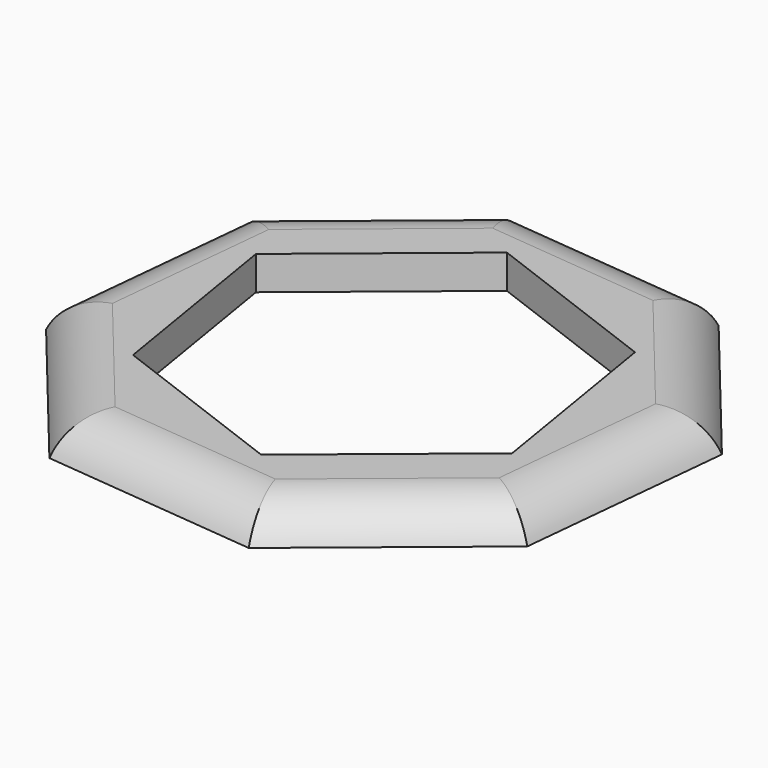
from build123d import *

# Parameters (mm, degrees)
F1_DEPTH     = 3
F2_T1_DEPTH  = 42.25719254
F2_T3_DEPTH  = 42.25719254
F2_T5_DEPTH  = 42.25719254
F2_T7_DEPTH  = 42.25719254
F2_T9_DEPTH  = 42.25719254
F2_T11_DEPTH = 42.25719254
F2_T13_DEPTH = 42.25719254
F2_T15_DEPTH = 42.25719254


# Not quite as in the source:
# - a fillet or chamfer that OpenCascade refuses, or shapes differently, is made with other operations: its cross-section is extruded or revolved along the edge and cut away or added


with BuildPart() as f1:
    # F0 (on Top) → F1 (new body)
    with BuildSketch(Plane.XY):
        Polygon((-56.6940829158, -6.0690771788), (-41.7333427947, 6.1938238515), (-39.825682479, 25.4438451183), (-52.0885835093, 40.4045852394), (-71.3386047761, 42.3122455551), (-86.2993448973, 30.0493445247), (-88.2070052129, 10.7993232579), (-75.9441041826, -4.1614168632), align=None)
        Polygon((-77.4948558278, 7.0736241854), (-80.3234138592, 24.2703379682), (-66.8449018774, 35.318297971), (-50.5378318641, 29.1695441909), (-47.7092738327, 11.972830408), (-61.1877858145, 0.9248704053), align=None, mode=Mode.SUBTRACT)
    extrude(amount=F1_DEPTH)

    # F2: fillet of radius 5 on 8 edges, made by hand

    # F2_s2 → F2_t1 (cut)
    with BuildSketch(Plane(origin=(-44.1465389595, 4.3748835016, 0), x_dir=(0, 0, 1), z_dir=(-0.9951255548, 0.0986160744, 0))):
        with BuildLine():
            ThreePointArc((0, 35.0708636755), (2.1833001327, 33.2269007681), (3, 30.4882879806))
            Line((3, 30.4882879806), (3, 35.0708636755))
            Line((3, 35.0708636755), (0, 35.0708636755))
        make_face()
    extrude(amount=F2_T1_DEPTH, mode=Mode.SUBTRACT)

    # F2_s4 → F2_t3 (cut)
    with BuildSketch(Plane(origin=(-13.0651926295, -10.709173668, 0), x_dir=(0, 0, 1), z_dir=(-0.7733921229, -0.633927933, 0))):
        with BuildLine():
            ThreePointArc((0, 77.9474916828), (2.1833001327, 76.1035287753), (3, 73.3649159878))
            Line((3, 73.3649159878), (3, 77.9474916828))
            Line((3, 77.9474916828), (0, 77.9474916828))
        make_face()
    extrude(amount=F2_T3_DEPTH, mode=Mode.SUBTRACT)

    # F2_s6 → F2_t5 (cut)
    with BuildSketch(Plane(origin=(3.2394204217, 32.6886875499, 0), x_dir=(0, 0, 1), z_dir=(-0.0986160744, -0.9951255548, 0))):
        with BuildLine():
            ThreePointArc((0, 88.8420318681), (2.1833001327, 86.9980689606), (3, 84.2594561731))
            Line((3, 84.2594561731), (3, 88.8420318681))
            Line((3, 88.8420318681), (0, 88.8420318681))
        make_face()
    extrude(amount=F2_T5_DEPTH, mode=Mode.SUBTRACT)

    # F2_s8 → F2_t7 (cut)
    with BuildSketch(Plane(origin=(-48.0044686533, 58.5654551398, 0), x_dir=(0, 0, 1), z_dir=(0.633927933, -0.7733921229, 0))):
        with BuildLine():
            ThreePointArc((0, 61.3726103468), (2.1833001327, 59.5286474393), (3, 56.7900346518))
            Line((3, 56.7900346518), (3, 61.3726103468))
            Line((3, 61.3726103468), (0, 61.3726103468))
        make_face()
    extrude(amount=F2_T7_DEPTH, mode=Mode.SUBTRACT)

    # F2_s10 → F2_t9 (cut)
    with BuildSketch(Plane(origin=(-86.1977511311, 8.5421219464, 0), x_dir=(0, 0, 1), z_dir=(0.9951255548, -0.0986160744, 0))):
        with BuildLine():
            ThreePointArc((0, 11.6304416954), (2.1833001327, 9.786478788), (3, 7.0478660005))
            Line((3, 7.0478660005), (3, 11.6304416954))
            Line((3, 11.6304416954), (0, 11.6304416954))
        make_face()
    extrude(amount=F2_T9_DEPTH, mode=Mode.SUBTRACT)

    # F2_s12 → F2_t11 (cut)
    with BuildSketch(Plane(origin=(-45.7465724763, -37.4971883885, 0), x_dir=(0, 0, 1), z_dir=(0.7733921229, 0.633927933, 0))):
        with BuildLine():
            ThreePointArc((0, -31.2461863118), (2.1833001327, -33.0901492192), (3, -35.8287620068))
            Line((3, -35.8287620068), (3, -31.2461863118))
            Line((3, -31.2461863118), (0, -31.2461863118))
        make_face()
    extrude(amount=F2_T11_DEPTH, mode=Mode.SUBTRACT)

    # F2_s14 → F2_t13 (cut)
    with BuildSketch(Plane(origin=(-0.927818023, -9.3625246217, 0), x_dir=(0, 0, 1), z_dir=(0.0986160744, 0.9951255548, 0))):
        with BuildLine():
            ThreePointArc((0, -42.1407264971), (2.1833001327, -43.9846894046), (3, -46.7233021921))
            Line((3, -46.7233021921), (3, -42.1407264971))
            Line((3, -42.1407264971), (0, -42.1407264971))
        make_face()
    extrude(amount=F2_T13_DEPTH, mode=Mode.SUBTRACT)

    # F2_s16 → F2_t15 (cut)
    with BuildSketch(Plane(origin=(-21.2164539328, 25.884075293, 0), x_dir=(0, 0, 1), z_dir=(-0.633927933, 0.7733921229, 0))):
        with BuildLine():
            ThreePointArc((0, -14.6713049758), (2.1833001327, -16.5152678832), (3, -19.2538806708))
            Line((3, -19.2538806708), (3, -14.6713049758))
            Line((3, -14.6713049758), (0, -14.6713049758))
        make_face()
    extrude(amount=F2_T15_DEPTH, mode=Mode.SUBTRACT)


solid = f1.part
